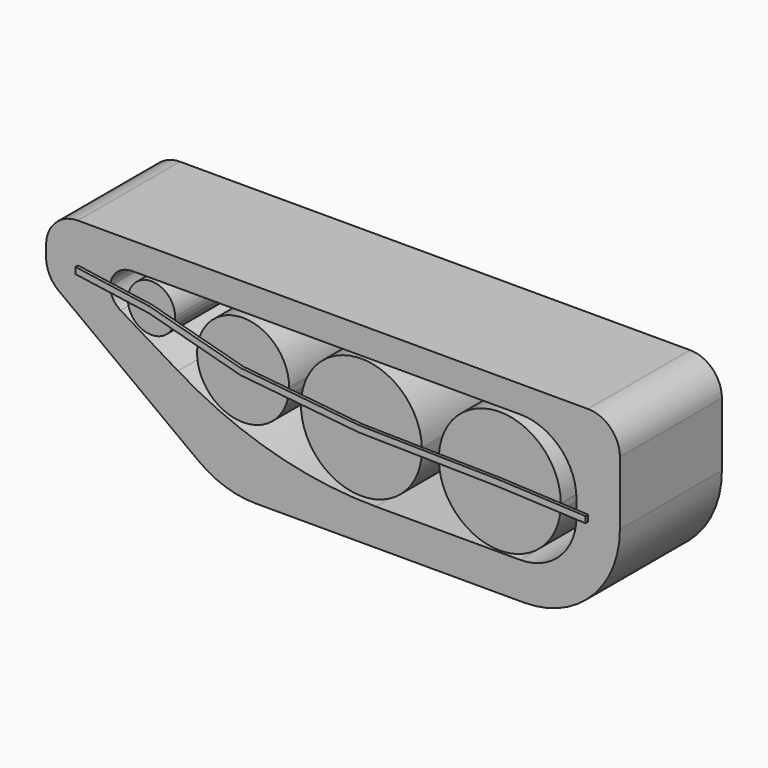
from build123d import *

# Parameters (mm, degrees)
F1_DEPTH    = 101.6
F2_R        = 25.4
F3_R        = 76.2
F4_R        = 25.4
F5_T1_DEPTH = 101.6
F6_R        = 44.7643478735
F7_R        = 304.8
F9_DEPTH    = 101.6
F10_DEPTH   = 2.54
F12_DEPTH   = 2.54


# Not quite as in the source:
# - a fillet or chamfer that OpenCascade refuses, or shapes differently, is made with other operations: its cross-section is extruded or revolved along the edge and cut away or added
# - a feature names something its author has since deleted; it is built from what else it names


with BuildPart() as f1:
    # F0 (on Front) → F1 (new body)
    with BuildSketch(Plane.XZ):
        Polygon((228.6, -76.2), (228.6, 76.2), (-228.6, 76.2), (-228.6, 29.4590149546), (-86.9704671455, -76.2), align=None)
        Polygon((-50.8129218496, -47.2383520842), (-177.8, 29.4590149546), (-177.8, 54.8590149546), (194.0227749825, 54.8590149546), (194.0227749825, -47.2383520842), align=None, mode=Mode.SUBTRACT)
    extrude(amount=F1_DEPTH)

    # F2
    f2_edges = [f1.edges().sort_by_distance(p)[0] for p in [
        (-228.6, -50.8, 76.2),
        (-228.6, -50.8, 29.459015),
    ]]
    fillet(f2_edges, radius=F2_R)

    # F3
    f3_edges = [f1.edges().sort_by_distance(p)[0] for p in [
        (-86.970467, -50.8, -76.2),
        (228.6, -50.8, -76.2),
    ]]
    fillet(f3_edges, radius=F3_R)

    # F4
    f4_edges = [f1.edges().sort_by_distance(p)[0] for p in [
        (228.6, -50.8, 76.2),
    ]]
    fillet(f4_edges, radius=F4_R)

    # F5: fillet of radius 17.78 on 2 edges, made by hand

    # F5_s2 → F5_t1 (join)
    with BuildSketch(Plane.XZ):
        with BuildLine():
            ThreePointArc((-169.2122093999, 24.2721806932), (-175.5049262693, 30.7540427919), (-177.8, 39.4916316146))
            Line((-177.8, 39.4916316146), (-177.8, 29.4590149546))
            Line((-177.8, 29.4590149546), (-169.2122093999, 24.2721806932))
        make_face()
        with BuildLine():
            ThreePointArc((-177.8, 37.0790149546), (-172.5923585695, 49.6513735241), (-160.02, 54.8590149546))
            Line((-160.02, 54.8590149546), (-177.8, 54.8590149546))
            Line((-177.8, 54.8590149546), (-177.8, 37.0790149546))
        make_face()
    extrude(amount=F5_T1_DEPTH)

    # F6
    f6_edges = [f1.edges().sort_by_distance(p)[0] for p in [
        (194.022775, -50.8, -47.238352),
        (194.022775, -50.8, 54.859015),
    ]]
    fillet(f6_edges, radius=F6_R)

    # F7
    f7_edges = [f1.edges().sort_by_distance(p)[0] for p in [
        (-50.812922, -50.8, -47.238352),
    ]]
    fillet(f7_edges, radius=F7_R)


with BuildPart() as f9:
    # F8 (on face) → F9 (new body)
    with BuildSketch(Plane.XZ.offset(101.6)):
        with BuildLine():
            ThreePointArc((181.5579526246, 2.7030038423), (181.5575706981, 2.8957391669), (181.5564249247, 3.0884714642))
            Line((181.5564249247, 3.0884714642), (132.9267988621, 5.2430038423))
            Line((132.9267988621, 5.2430038423), (84.4128365038, 6.0771070674))
            ThreePointArc((84.4128365038, 6.0771070674), (84.3028312187, 3.5389983943), (84.3255215946, 0.9986082775))
            Line((84.3255215946, 0.9986082775), (132.9267988621, 0.1630038423))
            Line((132.9267988621, 0.1630038423), (181.3317967881, -1.981576401))
            ThreePointArc((181.3317967881, -1.981576401), (181.5013807609, 0.3579857976), (181.5579526246, 2.7030038423))
        make_face()
        with BuildLine():
            Line((132.9267988621, 5.2430038423), (181.5564249247, 3.0884714642))
            ThreePointArc((181.5564249247, 3.0884714642), (134.4222353253, 51.3111593931), (84.4128365038, 6.0771070674))
            Line((84.4128365038, 6.0771070674), (132.9267988621, 5.2430038423))
        make_face()
        with BuildLine():
            Line((132.9267988621, 0.1630038423), (84.3255215946, 0.9986082775))
            ThreePointArc((84.3255215946, 0.9986082775), (131.4334782085, -45.9052167557), (181.3317967881, -1.981576401))
            Line((181.3317967881, -1.981576401), (132.9267988621, 0.1630038423))
        make_face()
    extrude(amount=-F9_DEPTH)


with BuildPart() as f9b:
    # F8 (on face) → F9, piece 2 (new body)
    with BuildSketch(Plane.XZ.offset(101.6)):
        with BuildLine():
            ThreePointArc((-24.933795283, 11.9335457727), (-25.2529707533, 9.4256839495), (-25.4401728054, 6.904533558))
            Line((-25.4401728054, 6.904533558), (22.6892231991, 2.0583245484))
            Line((22.6892231991, 2.0583245484), (70.7560995281, 1.231908098))
            ThreePointArc((70.7560995281, 1.231908098), (70.8443963799, 2.9140871326), (70.8738406589, 4.5983245484))
            ThreePointArc((70.8738406589, 4.5983245484), (70.866233503, 5.4545008872), (70.8434144374, 6.3104068879))
            Line((70.8434144374, 6.3104068879), (22.6892231991, 7.1383245484))
            Line((22.6892231991, 7.1383245484), (-24.933795283, 11.9335457727))
        make_face()
        with BuildLine():
            ThreePointArc((70.8434144374, 6.3104068879), (25.5133086889, 52.7001114268), (-24.933795283, 11.9335457727))
            Line((-24.933795283, 11.9335457727), (22.6892231991, 7.1383245484))
            Line((22.6892231991, 7.1383245484), (70.8434144374, 6.3104068879))
        make_face()
        with BuildLine():
            Line((22.6892231991, 2.0583245484), (-25.4401728054, 6.904533558))
            ThreePointArc((-25.4401728054, 6.904533558), (19.8527382123, -43.5027327442), (70.7560995281, 1.231908098))
            Line((70.7560995281, 1.231908098), (22.6892231991, 2.0583245484))
        make_face()
    extrude(amount=-F9_DEPTH)


with BuildPart() as f9c:
    # F8 (on face) → F9, piece 3 (new body)
    with BuildSketch(Plane.XZ.offset(101.6)):
        with BuildLine():
            Line((-71.6374335136, 16.6361934509), (-106.3043915588, 26.0207271152))
            ThreePointArc((-106.3043915588, 26.0207271152), (-107.0242596832, 23.6755993229), (-107.5856804463, 21.2875789701))
            Line((-107.5856804463, 21.2875789701), (-71.6374335136, 11.5561934509))
            Line((-71.6374335136, 11.5561934509), (-35.5013362705, 7.9176046763))
            ThreePointArc((-35.5013362705, 7.9176046763), (-35.1613745589, 10.4233735068), (-34.994958748, 12.9466168909))
            Line((-34.994958748, 12.9466168909), (-71.6374335136, 16.6361934509))
        make_face()
        with BuildLine():
            ThreePointArc((-34.9769304727, 14.0961934509), (-65.5924205947, 50.2548757005), (-106.3043915588, 26.0207271152))
            Line((-106.3043915588, 26.0207271152), (-71.6374335136, 16.6361934509))
            Line((-71.6374335136, 16.6361934509), (-34.994958748, 12.9466168909))
            ThreePointArc((-34.994958748, 12.9466168909), (-34.9814378186, 13.521334493), (-34.9769304727, 14.0961934509))
        make_face()
        with BuildLine():
            Line((-71.6374335136, 11.5561934509), (-107.5856804463, 21.2875789701))
            ThreePointArc((-107.5856804463, 21.2875789701), (-78.3230804598, -21.9495359512), (-35.5013362705, 7.9176046763))
            Line((-35.5013362705, 7.9176046763), (-71.6374335136, 11.5561934509))
        make_face()
    extrude(amount=-F9_DEPTH)


with BuildPart() as f9d:
    # F8 (on face) → F9, piece 4 (new body)
    with BuildSketch(Plane.XZ.offset(101.6)):
        with BuildLine():
            Line((-144.6040853896, 36.3886620699), (-162.7251657845, 38.9712052824))
            ThreePointArc((-162.7251657845, 38.9712052824), (-163.2469093716, 36.5055620718), (-163.4347349564, 33.9923302158))
            Line((-163.4347349564, 33.9923302158), (-144.6040853896, 31.3086620699))
            Line((-144.6040853896, 31.3086620699), (-127.2224929369, 26.6033706712))
            ThreePointArc((-127.2224929369, 26.6033706712), (-126.4271303203, 28.9280616948), (-125.9412040494, 31.3365188163))
            Line((-125.9412040494, 31.3365188163), (-144.6040853896, 36.3886620699))
        make_face()
        with BuildLine():
            ThreePointArc((-125.9412040494, 31.3365188163), (-125.8150139618, 32.5897742577), (-125.7728877738, 33.8486620699))
            ThreePointArc((-125.7728877738, 33.8486620699), (-142.0183207333, 52.501485577), (-162.7251657845, 38.9712052824))
            Line((-162.7251657845, 38.9712052824), (-144.6040853896, 36.3886620699))
            Line((-144.6040853896, 36.3886620699), (-125.9412040494, 31.3365188163))
        make_face()
        with BuildLine():
            Line((-144.6040853896, 31.3086620699), (-163.4347349564, 33.9923302158))
            ThreePointArc((-163.4347349564, 33.9923302158), (-148.3689389615, 15.3976490564), (-127.2224929369, 26.6033706712))
            Line((-127.2224929369, 26.6033706712), (-144.6040853896, 31.3086620699))
        make_face()
    extrude(amount=-F9_DEPTH)


with BuildPart() as f10:
    # F8 (on face) → F10 (new body)
    with BuildSketch(Plane.XZ.offset(101.6)):
        with BuildLine():
            ThreePointArc((-24.933795283, 11.9335457727), (-25.2529707533, 9.4256839495), (-25.4401728054, 6.904533558))
            Line((-25.4401728054, 6.904533558), (22.6892231991, 2.0583245484))
            Line((22.6892231991, 2.0583245484), (70.7560995281, 1.231908098))
            ThreePointArc((70.7560995281, 1.231908098), (70.8443963799, 2.9140871326), (70.8738406589, 4.5983245484))
            ThreePointArc((70.8738406589, 4.5983245484), (70.866233503, 5.4545008872), (70.8434144374, 6.3104068879))
            Line((70.8434144374, 6.3104068879), (22.6892231991, 7.1383245484))
            Line((22.6892231991, 7.1383245484), (-24.933795283, 11.9335457727))
        make_face()
        with BuildLine():
            ThreePointArc((-34.994958748, 12.9466168909), (-35.1613745589, 10.4233735068), (-35.5013362705, 7.9176046763))
            Line((-35.5013362705, 7.9176046763), (-25.4401728054, 6.904533558))
            ThreePointArc((-25.4401728054, 6.904533558), (-25.2529707533, 9.4256839495), (-24.933795283, 11.9335457727))
            Line((-24.933795283, 11.9335457727), (-34.994958748, 12.9466168909))
        make_face()
        with BuildLine():
            Line((-71.6374335136, 16.6361934509), (-106.3043915588, 26.0207271152))
            ThreePointArc((-106.3043915588, 26.0207271152), (-107.0242596832, 23.6755993229), (-107.5856804463, 21.2875789701))
            Line((-107.5856804463, 21.2875789701), (-71.6374335136, 11.5561934509))
            Line((-71.6374335136, 11.5561934509), (-35.5013362705, 7.9176046763))
            ThreePointArc((-35.5013362705, 7.9176046763), (-35.1613745589, 10.4233735068), (-34.994958748, 12.9466168909))
            Line((-34.994958748, 12.9466168909), (-71.6374335136, 16.6361934509))
        make_face()
        with BuildLine():
            ThreePointArc((70.8738406589, 4.5983245484), (70.8443963799, 2.9140871326), (70.7560995281, 1.231908098))
            Line((70.7560995281, 1.231908098), (84.3255215946, 0.9986082775))
            ThreePointArc((84.3255215946, 0.9986082775), (84.3028312187, 3.5389983943), (84.4128365038, 6.0771070674))
            Line((84.4128365038, 6.0771070674), (70.8434144374, 6.3104068879))
            ThreePointArc((70.8434144374, 6.3104068879), (70.866233503, 5.4545008872), (70.8738406589, 4.5983245484))
        make_face()
        with BuildLine():
            ThreePointArc((181.5579526246, 2.7030038423), (181.5575706981, 2.8957391669), (181.5564249247, 3.0884714642))
            Line((181.5564249247, 3.0884714642), (132.9267988621, 5.2430038423))
            Line((132.9267988621, 5.2430038423), (84.4128365038, 6.0771070674))
            ThreePointArc((84.4128365038, 6.0771070674), (84.3028312187, 3.5389983943), (84.3255215946, 0.9986082775))
            Line((84.3255215946, 0.9986082775), (132.9267988621, 0.1630038423))
            Line((132.9267988621, 0.1630038423), (181.3317967881, -1.981576401))
            ThreePointArc((181.3317967881, -1.981576401), (181.5013807609, 0.3579857976), (181.5579526246, 2.7030038423))
        make_face()
        with BuildLine():
            Line((194.0227749825, -2.4740042106), (194.0227749825, 2.5361506464))
            Line((194.0227749825, 2.5361506464), (181.5564249247, 3.0884714642))
            ThreePointArc((181.5564249247, 3.0884714642), (181.5575706981, 2.8957391669), (181.5579526246, 2.7030038423))
            ThreePointArc((181.5579526246, 2.7030038423), (181.5013807609, 0.3579857976), (181.3317967881, -1.981576401))
            Line((181.3317967881, -1.981576401), (194.022720497, -2.5438469397))
            ThreePointArc((194.022720497, -2.5438469397), (194.0227613611, -2.5089255858), (194.0227749825, -2.4740042106))
        make_face()
        with BuildLine():
            Line((-144.6040853896, 36.3886620699), (-162.7251657845, 38.9712052824))
            ThreePointArc((-162.7251657845, 38.9712052824), (-163.2469093716, 36.5055620718), (-163.4347349564, 33.9923302158))
            Line((-163.4347349564, 33.9923302158), (-144.6040853896, 31.3086620699))
            Line((-144.6040853896, 31.3086620699), (-127.2224929369, 26.6033706712))
            ThreePointArc((-127.2224929369, 26.6033706712), (-126.4271303203, 28.9280616948), (-125.9412040494, 31.3365188163))
            Line((-125.9412040494, 31.3365188163), (-144.6040853896, 36.3886620699))
        make_face()
        with BuildLine():
            Line((-106.3043915588, 26.0207271152), (-125.9412040494, 31.3365188163))
            ThreePointArc((-125.9412040494, 31.3365188163), (-126.4271303203, 28.9280616948), (-127.2224929369, 26.6033706712))
            Line((-127.2224929369, 26.6033706712), (-107.5856804463, 21.2875789701))
            ThreePointArc((-107.5856804463, 21.2875789701), (-107.0242596832, 23.6755993229), (-106.3043915588, 26.0207271152))
        make_face()
        with BuildLine():
            ThreePointArc((-163.4347349564, 33.9923302158), (-163.2469093716, 36.5055620718), (-162.7251657845, 38.9712052824))
            Line((-162.7251657845, 38.9712052824), (-177.3496436399, 41.0554268187))
            ThreePointArc((-177.3496436399, 41.0554268187), (-177.6089554365, 39.678446941), (-177.7590309829, 38.2853232846))
            ThreePointArc((-177.7590309829, 38.2853232846), (-177.642814272, 37.1326451513), (-177.4517771113, 35.9899824687))
            Line((-177.4517771113, 35.9899824687), (-163.4347349564, 33.9923302158))
        make_face()
        with BuildLine():
            ThreePointArc((-177.7590309829, 38.2853232846), (-177.6089554365, 39.678446941), (-177.3496436399, 41.0554268187))
            Line((-177.3496436399, 41.0554268187), (-203.2, 44.7395152341))
            Line((-203.2, 44.7395152341), (-203.2, 42.1995152341))
            Line((-203.2, 42.1995152341), (-203.2, 39.6595152341))
            Line((-203.2, 39.6595152341), (-177.4517771113, 35.9899824687))
            ThreePointArc((-177.4517771113, 35.9899824687), (-177.642814272, 37.1326451513), (-177.7590309829, 38.2853232846))
        make_face()
        with BuildLine():
            Line((203.2, 2.1295542967), (194.0227749825, 2.5361506464))
            Line((194.0227749825, 2.5361506464), (194.0227749825, -2.4740042106))
            ThreePointArc((194.0227749825, -2.4740042106), (194.0227613611, -2.5089255858), (194.022720497, -2.5438469397))
            Line((194.022720497, -2.5438469397), (203.2, -2.9504457033))
            Line((203.2, -2.9504457033), (203.2, -0.4104457033))
            Line((203.2, -0.4104457033), (203.2, 2.1295542967))
        make_face()
    extrude(amount=F10_DEPTH)


with BuildPart() as f12:
    # F11 (on face) → F12 (new body)
    with BuildSketch(Plane(origin=(0, 0, 0), x_dir=(-1, 0, 0), z_dir=(0, 1, 0))):
        with BuildLine():
            Line((-135.4079395533, 5.2261864766), (-194.0227749825, 2.5366485965))
            Line((-194.0227749825, 2.5366485965), (-194.0227749825, -2.4740042106))
            ThreePointArc((-194.0227749825, -2.4740042106), (-194.0227435045, -2.5270907724), (-194.0226490705, -2.5801772595))
            Line((-194.0226490705, -2.5801772595), (-134.5681399107, 0))
            Line((-134.5681399107, 0), (-22.5686617196, 2.0149990451))
            Line((-22.5686617196, 2.0149990451), (71.4773535728, 11.5748010576))
            Line((71.4773535728, 11.5748010576), (144.7256356478, 31.3955061138))
            Line((144.7256356478, 31.3955061138), (177.4757826865, 36.1116832716))
            ThreePointArc((177.4757826865, 36.1116832716), (177.6509360226, 37.1941340701), (177.7590309829, 38.2853232846))
            ThreePointArc((177.7590309829, 38.2853232846), (177.6055562192, 39.7013445412), (177.3392307825, 41.1005376887))
            Line((177.3392307825, 41.1005376887), (144.6800976992, 36.4504270256))
            Line((144.6800976992, 36.4504270256), (71.608915925, 16.6399870068))
            Line((71.608915925, 16.6399870068), (-22.7780099958, 7.1439980529))
            Line((-22.7780099958, 7.1439980529), (-135.4079395533, 5.2261864766))
        make_face()
        with BuildLine():
            Line((203.2, 44.7826758027), (177.3392307825, 41.1005376887))
            ThreePointArc((177.3392307825, 41.1005376887), (177.6055562192, 39.7013445412), (177.7590309829, 38.2853232846))
            ThreePointArc((177.7590309829, 38.2853232846), (177.6509360226, 37.1941340701), (177.4757826865, 36.1116832716))
            Line((177.4757826865, 36.1116832716), (203.199505806, 39.8160219193))
            Line((203.199505806, 39.8160219193), (203.2, 44.7826758027))
        make_face()
        with BuildLine():
            Line((-194.0227749825, 2.5366485965), (-203.1785696745, 2.1165355574))
            Line((-203.1785696745, 2.1165355574), (-203.2696157694, -2.9814725276))
            Line((-203.2696157694, -2.9814725276), (-194.0226490705, -2.5801772595))
            ThreePointArc((-194.0226490705, -2.5801772595), (-194.0227435045, -2.5270907724), (-194.0227749825, -2.4740042106))
            Line((-194.0227749825, -2.4740042106), (-194.0227749825, 2.5366485965))
        make_face()
    extrude(amount=F12_DEPTH)


solid = Compound([f1.part, f9.part, f9b.part, f9c.part, f9d.part, f10.part, f12.part])
